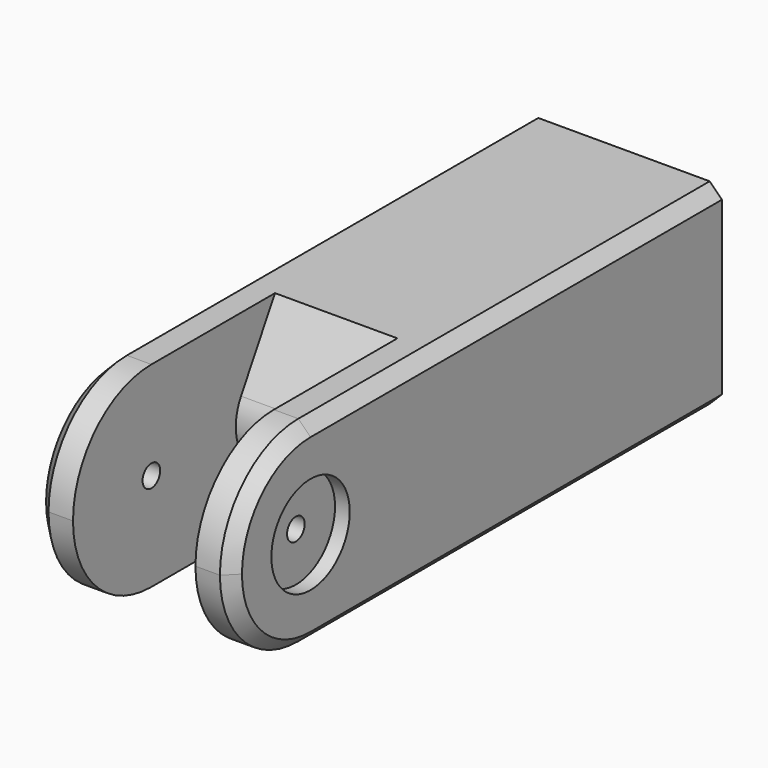
from build123d import *

# Parameters (mm, degrees)
F0_W      = 250
F0_H      = 80
F1_DEPTH  = 40
F2_R      = 39.99999
F4_DEPTH  = 25
F5_R      = 20
F6_SIZE   = 5
F7_R      = 4.5
F8_DEPTH  = 80.001
F9_R      = 20
F10_DEPTH = 6


# Not quite as in the source:
# - a fillet or chamfer is up to 0.001 mm smaller than in the source, because OpenCascade refuses the exact size
# - a pattern or mirror of a feature is missing from the dataset's text; its kind, count and spacing are read off the source's solid


with BuildPart() as f1:
    # F0 (on Right) → F1 (new body, symmetric)
    with BuildSketch(Plane.YZ):
        Rectangle(F0_W, F0_H)
    extrude(amount=F1_DEPTH, both=True)

    # F2 (radius 40 in the source; OpenCascade refuses exactly that, so slightly less here)
    f2_edges = [f1.edges().sort_by_distance(p)[0] for p in [
        (0, -125, 40),
        (0, -125, -40),
    ]]
    fillet(f2_edges, radius=F2_R)

    # F3 (on Right) → F4 (cut, symmetric)
    with BuildSketch(Plane.YZ):
        Polygon((-21.9059892324, -40), (-45, 0), (-21.9059892324, 40), (-155.967399478, 40), (-155.967399478, -40), align=None)
    extrude(amount=F4_DEPTH, both=True, mode=Mode.SUBTRACT)

    # F5
    f5_edges = [f1.edges().sort_by_distance(p)[0] for p in [
        (0, -45, 0),
    ]]
    fillet(f5_edges, radius=F5_R)

    # F6
    f6_edges = [f1.edges().sort_by_distance(p)[0] for p in [
        (40, 19.999995, 40),
        (-40, 19.999995, 40),
        (40, -113.284274, 28.284274),
        (40, 19.999995, -40),
        (-40, 19.999995, -40),
        (40, -125, 0),
        (40, -113.284274, -28.284274),
        (-40, -113.284274, 28.284274),
        (-40, -125, 0),
        (-40, -113.284274, -28.284274),
    ]]
    chamfer(f6_edges, length=F6_SIZE)

    # F7 (on face) → F8 (cut, through all)
    with BuildSketch(Plane.YZ.offset(40)):
        with Locations((-85, 0)):
            Circle(F7_R)
    extrude(amount=-F8_DEPTH, mode=Mode.SUBTRACT)

    # F9 (on face) → F10 (cut)
    with BuildSketch(Plane.YZ.offset(40)):
        with Locations((-85, 0)):
            Circle(F9_R)
    f10 = extrude(amount=-F10_DEPTH, mode=Mode.SUBTRACT)

    # F10_copies: F10 across plane
    add(f10.mirror(Plane(origin=(0, 0, 0), x_dir=(0, 0, -1), z_dir=(-1, 0, 0))), mode=Mode.SUBTRACT)


solid = f1.part
